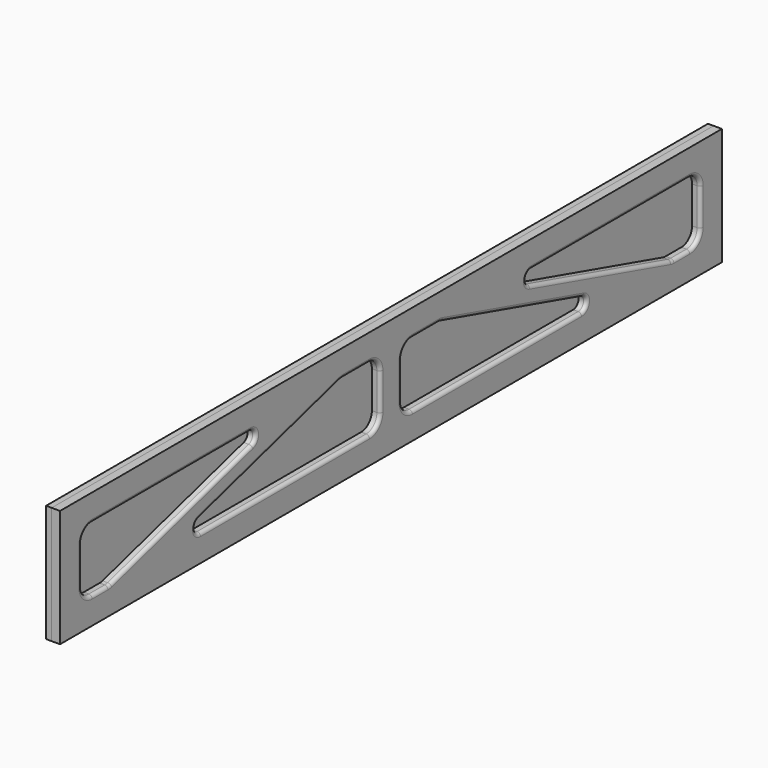
from build123d import *

# Parameters (mm, degrees)
F2_W     = 939.8
F2_H     = 133.35
F3_DEPTH = 9.525
F4_R     = 15.24
F5_R     = 7.62
F6_R     = 3.81
F7_W     = 939.8
F7_H     = 133.35
F8_DEPTH = 6.35


with BuildPart() as f3:
    # F2 (on face) → F3 (new body)
    with BuildSketch(Plane(origin=(247.65, 0, 0), x_dir=(0, -1, 0), z_dir=(-1, 0, 0))):
        with Locations((-469.9, 66.675)):
            Rectangle(F2_W, F2_H)
        Polygon((-909.32, 30.48), (-909.32, 102.87), (-614.5213290809, 102.87), (-869.6099005094, 30.48), align=None, mode=Mode.SUBTRACT)
        Polygon((-540.0900994906, 102.87), (-485.14, 102.87), (-485.14, 30.48), (-795.1786709191, 30.48), align=None, mode=Mode.SUBTRACT)
        Polygon((-399.7099005094, 102.87), (-144.6213290809, 30.48), (-454.66, 30.48), (-454.66, 102.87), align=None, mode=Mode.SUBTRACT)
        Polygon((-30.48, 102.87), (-30.48, 30.48), (-70.1900994906, 30.48), (-325.2786709191, 102.87), align=None, mode=Mode.SUBTRACT)
    extrude(amount=F3_DEPTH)

    # F4
    f4_edges = [f3.edges().sort_by_distance(p)[0] for p in [
        (242.8875, 399.709901, 102.87),
        (242.8875, 454.66, 102.87),
        (242.8875, 454.66, 30.48),
        (242.8875, 30.48, 30.48),
        (242.8875, 30.48, 102.87),
        (242.8875, 70.190099, 30.48),
        (242.8875, 540.090099, 102.87),
        (242.8875, 485.14, 102.87),
        (242.8875, 485.14, 30.48),
        (242.8875, 909.32, 102.87),
        (242.8875, 909.32, 30.48),
        (242.8875, 869.609901, 30.48),
    ]]
    fillet(f4_edges, radius=F4_R)

    # F5
    f5_edges = [f3.edges().sort_by_distance(p)[0] for p in [
        (242.8875, 144.621329, 30.48),
        (242.8875, 614.521329, 102.87),
        (242.8875, 795.178671, 30.48),
        (242.8875, 325.278671, 102.87),
    ]]
    fillet(f5_edges, radius=F5_R)

    # F6
    f6_edges = [f3.edges().sort_by_distance(p)[0] for p in [
        (247.65, 158.117766, 102.87),
        (247.65, 297.487035, 73.860808),
        (247.65, 519.174767, 102.87),
        (247.65, 781.682234, 102.87),
    ]]
    fillet(f6_edges, radius=F6_R)


with BuildPart() as f8:
    # F7 (on face) → F8 (new body)
    with BuildSketch(Plane(origin=(238.125, 0, 0), x_dir=(0, -1, 0), z_dir=(-1, 0, 0))):
        with Locations((-469.9, 66.675)):
            Rectangle(F7_W, F7_H)
    extrude(amount=F8_DEPTH)


solid = Compound([f3.part, f8.part])
